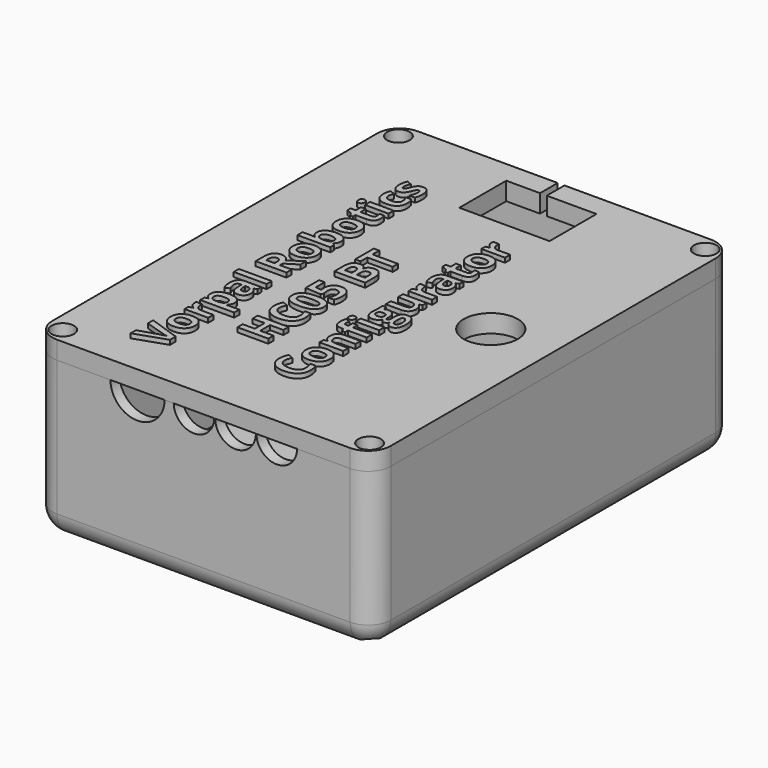
from build123d import *

# Parameters (mm, degrees)
F0_W          = 75
F0_H          = 100
F0_R          = 2.5
F0_R_2        = 1.6
F1_DEPTH      = 35
F2_T          = -2.5
F3_T1_DEPTH   = 42.5
F3_T3_DEPTH   = 65
F3_T5_DEPTH   = 90
F3_S9_W       = 5
F3_S9_H       = 5
F3_T10_DEPTH  = 5
F3_S15_W      = 5
F3_S15_H      = 5
F3_T16_DEPTH  = 5
F3_S21_W      = 5
F3_S21_H      = 5
F3_T22_DEPTH  = 5
F3_S27_W      = 5
F3_S27_H      = 5
F3_T28_DEPTH  = 5
F4_R          = 6
F4_R_2        = 4.5
F5_DEPTH      = 25
F6_DEPTH      = 4
F7_R          = 5
F8_R          = 6
F9_DEPTH      = 39.0010001
F10_TEXT_SIZE = 9.573958832
F11_DEPTH     = 1


# Not quite as in the source:
# - a fillet or chamfer that OpenCascade refuses, or shapes differently, is made with other operations: its cross-section is extruded or revolved along the edge and cut away or added
# - Text() gives the source's letters only with a copy of the font that has no kerning and outlines rounded to 1/6400 em; it was checked with that copy


with BuildPart() as f1:
    # F0 (on Top) → F1 (new body)
    with BuildSketch(Plane.XY):
        Rectangle(F0_W, F0_H)
        with Locations((-34, -46.5)):
            Circle(F0_R, mode=Mode.SUBTRACT)
        with Locations((34, -46.5)):
            Circle(F0_R, mode=Mode.SUBTRACT)
        with Locations((-34, 46.5)):
            Circle(F0_R, mode=Mode.SUBTRACT)
        with Locations((34, 46.5)):
            Circle(F0_R, mode=Mode.SUBTRACT)
        with Locations((-34, 46.5)):
            Circle(F0_R)
        with Locations((-34, 46.5)):
            Circle(F0_R_2, mode=Mode.SUBTRACT)
        with Locations((34, 46.5)):
            Circle(F0_R)
        with Locations((34, 46.5)):
            Circle(F0_R_2, mode=Mode.SUBTRACT)
        with Locations((-34, -46.5)):
            Circle(F0_R)
        with Locations((-34, -46.5)):
            Circle(F0_R_2, mode=Mode.SUBTRACT)
        with Locations((34, -46.5)):
            Circle(F0_R)
        with Locations((34, -46.5)):
            Circle(F0_R_2, mode=Mode.SUBTRACT)
    extrude(amount=-F1_DEPTH)

    # F2
    f2_openings = [f1.faces().sort_by_distance(p)[0] for p in [
        (0, 0, 0),
    ]]
    offset(amount=F2_T, openings=f2_openings)

    # F3: fillet of radius 5 on 8 edges, made by hand

    # F3_s2 → F3_t1 (cut)
    with BuildSketch(Plane.XY.offset(-30)):
        with BuildLine():
            ThreePointArc((-32.5, -50), (-36.0355339059, -48.5355339059), (-37.5, -45))
            Line((-37.5, -45), (-37.5, -50))
            Line((-37.5, -50), (-32.5, -50))
        make_face()
        with BuildLine():
            ThreePointArc((32.5, -50), (36.0355339059, -48.5355339059), (37.5, -45))
            Line((37.5, -45), (37.5, -50))
            Line((37.5, -50), (32.5, -50))
        make_face()
        with BuildLine():
            ThreePointArc((37.5, 45), (36.0355339059, 48.5355339059), (32.5, 50))
            Line((32.5, 50), (37.5, 50))
            Line((37.5, 50), (37.5, 45))
        make_face()
        with BuildLine():
            ThreePointArc((-32.5, 50), (-36.0355339059, 48.5355339059), (-37.5, 45))
            Line((-37.5, 45), (-37.5, 50))
            Line((-37.5, 50), (-32.5, 50))
        make_face()
    extrude(amount=F3_T1_DEPTH, mode=Mode.SUBTRACT)

    # F3_s4 → F3_t3 (cut)
    with BuildSketch(Plane.YZ.offset(-32.5)):
        with BuildLine():
            ThreePointArc((50, -30), (48.5355339059, -33.5355339059), (45, -35))
            Line((45, -35), (50, -35))
            Line((50, -35), (50, -30))
        make_face()
        with BuildLine():
            ThreePointArc((-50, -30), (-48.5355339059, -33.5355339059), (-45, -35))
            Line((-45, -35), (-50, -35))
            Line((-50, -35), (-50, -30))
        make_face()
    extrude(amount=F3_T3_DEPTH, mode=Mode.SUBTRACT)

    # F3_s6 → F3_t5 (cut)
    with BuildSketch(Plane.XZ.offset(-45)):
        with BuildLine():
            ThreePointArc((-37.5, -30), (-36.0355339059, -33.5355339059), (-32.5, -35))
            Line((-32.5, -35), (-37.5, -35))
            Line((-37.5, -35), (-37.5, -30))
        make_face()
        with BuildLine():
            ThreePointArc((37.5, -30), (36.0355339059, -33.5355339059), (32.5, -35))
            Line((32.5, -35), (37.5, -35))
            Line((37.5, -35), (37.5, -30))
        make_face()
    extrude(amount=F3_T5_DEPTH, mode=Mode.SUBTRACT)


with BuildPart() as f3_tool8:
    # F3_s9 → F3_t10 (new body)
    with BuildSketch(Plane.XZ.offset(45)):
        with Locations((-35, -32.5)):
            Rectangle(F3_S9_W, F3_S9_H)
    extrude(amount=F3_T10_DEPTH)

    # F3_s11 → F3_t12 (revolve, cut)
    with BuildSketch(Plane(origin=(-32.5, -45, -30), x_dir=(0.7071067812, 0, 0.7071067812), z_dir=(0.7071067812, 0, -0.7071067812))):
        with BuildLine():
            ThreePointArc((0, -5), (5, 0), (0, 5))
            Line((0, 5), (0, -5))
        make_face()
    revolve(axis=Axis((-32.5, -45, -30), (0, -1, 0)), mode=Mode.SUBTRACT)


with BuildPart() as f1_1:
    add(f1.part)

    # F3_t7: cut F3_tool8
    add(f3_tool8.part, mode=Mode.SUBTRACT)


with BuildPart() as f3_tool14:
    # F3_s15 → F3_t16 (new body)
    with BuildSketch(Plane.XZ.offset(45)):
        with Locations((35, -32.5)):
            Rectangle(F3_S15_W, F3_S15_H)
    extrude(amount=F3_T16_DEPTH)

    # F3_s17 → F3_t18 (revolve, cut)
    with BuildSketch(Plane(origin=(32.5, -45, -30), x_dir=(-0.7071067812, 0, 0.7071067812), z_dir=(0.7071067812, 0, 0.7071067812))):
        with BuildLine():
            ThreePointArc((0, -5), (5, 0), (0, 5))
            Line((0, 5), (0, -5))
        make_face()
    revolve(axis=Axis((32.5, -45, -30), (0, -1, 0)), mode=Mode.SUBTRACT)


with BuildPart() as f1_2:
    add(f1_1.part)

    # F3_t13: cut F3_tool14
    add(f3_tool14.part, mode=Mode.SUBTRACT)


with BuildPart() as f3_tool20:
    # F3_s21 → F3_t22 (new body)
    with BuildSketch(Plane.YZ.offset(32.5)):
        with Locations((47.5, -32.5)):
            Rectangle(F3_S21_W, F3_S21_H)
    extrude(amount=F3_T22_DEPTH)

    # F3_s23 → F3_t24 (revolve, cut)
    with BuildSketch(Plane(origin=(32.5, 45, -30), x_dir=(0, -0.7071067812, 0.7071067812), z_dir=(0, 0.7071067812, 0.7071067812))):
        with BuildLine():
            ThreePointArc((0, -5), (5, 0), (0, 5))
            Line((0, 5), (0, -5))
        make_face()
    revolve(axis=Axis((32.5, 45, -30), (1, 0, 0)), mode=Mode.SUBTRACT)


with BuildPart() as f1_3:
    add(f1_2.part)

    # F3_t19: cut F3_tool20
    add(f3_tool20.part, mode=Mode.SUBTRACT)


with BuildPart() as f3_tool26:
    # F3_s27 → F3_t28 (new body)
    with BuildSketch(Plane.XZ.offset(-45)):
        with Locations((-35, -32.5)):
            Rectangle(F3_S27_W, F3_S27_H)
    extrude(amount=-F3_T28_DEPTH)

    # F3_s29 → F3_t30 (revolve, cut)
    with BuildSketch(Plane(origin=(-32.5, 45, -30), x_dir=(0.7071067812, 0, 0.7071067812), z_dir=(-0.7071067812, 0, 0.7071067812))):
        with BuildLine():
            ThreePointArc((0, -5), (5, 0), (0, 5))
            Line((0, 5), (0, -5))
        make_face()
    revolve(axis=Axis((-32.5, 45, -30), (0, 1, 0)), mode=Mode.SUBTRACT)


with BuildPart() as f1_4:
    add(f1_3.part)

    # F3_t25: cut F3_tool26
    add(f3_tool26.part, mode=Mode.SUBTRACT)

    # F4 (on face) → F5 (cut)
    with BuildSketch(Plane.XZ.offset(50)):
        with Locations((-14.6300764754, 0)):
            Circle(F4_R)
        with Locations((-2.1105410997, 0.0705600396)):
            Circle(F4_R_2)
        with Locations((7.0949820802, 0)):
            Circle(F4_R_2)
        with Locations((16.2307694554, 0)):
            Circle(F4_R_2)
    extrude(amount=-F5_DEPTH, mode=Mode.SUBTRACT)


with BuildPart() as f6:
    # F0 (on Top) → F6 (new body)
    with BuildSketch(Plane.XY):
        Rectangle(F0_W, F0_H)
        with Locations((-34, -46.5)):
            Circle(F0_R, mode=Mode.SUBTRACT)
        with Locations((34, -46.5)):
            Circle(F0_R, mode=Mode.SUBTRACT)
        with Locations((-34, 46.5)):
            Circle(F0_R, mode=Mode.SUBTRACT)
        with Locations((34, 46.5)):
            Circle(F0_R, mode=Mode.SUBTRACT)
    extrude(amount=F6_DEPTH)

    # F7
    f7_edges = [f6.edges().sort_by_distance(p)[0] for p in [
        (-37.5, -50, 2),
        (37.5, -50, 2),
        (37.5, 50, 2),
        (-37.5, 50, 2),
    ]]
    fillet(f7_edges, radius=F7_R)

    # F8 (on face) → F9 (cut, through all)
    with BuildSketch(Plane.XY.offset(4)):
        Polygon((-1.5, 45.1010205144), (-8.9890961349, 45.1010205144), (-8.9890961349, 32.1010205144), (11.0109038651, 32.1010205144), (11.0109038651, 45.1010205144), (0, 45.1010205144), (0, 53.6337606609), (-1.5, 53.6337606609), align=None)
        with Locations((23.6662887037, 0)):
            Circle(F8_R)
    extrude(amount=-F9_DEPTH, mode=Mode.SUBTRACT)

    # F10 (on face) → F11 (join)
    with BuildSketch(Plane.XY.offset(4)):
        with Locations(Location((-15.9792329988, -41.6472181678), (0, 0, 90))):
            Text('Vorpal Robotics', F10_TEXT_SIZE, font='Open Sans', font_style=FontStyle.BOLD, text_align=(TextAlign.LEFT, TextAlign.BOTTOM))
        with Locations(Location((-2.9586489873, -29.2085513415), (0, 0, 90))):
            Text('HC05 BT', F10_TEXT_SIZE, font='Open Sans', font_style=FontStyle.BOLD, text_align=(TextAlign.LEFT, TextAlign.BOTTOM))
        with Locations(Location((10.0619350242, -36.6717514373), (0, 0, 90))):
            Text('Configurator', F10_TEXT_SIZE, font='Open Sans', font_style=FontStyle.BOLD, text_align=(TextAlign.LEFT, TextAlign.BOTTOM))
    extrude(amount=F11_DEPTH)


solid = Compound([f1_4.part, f6.part])
